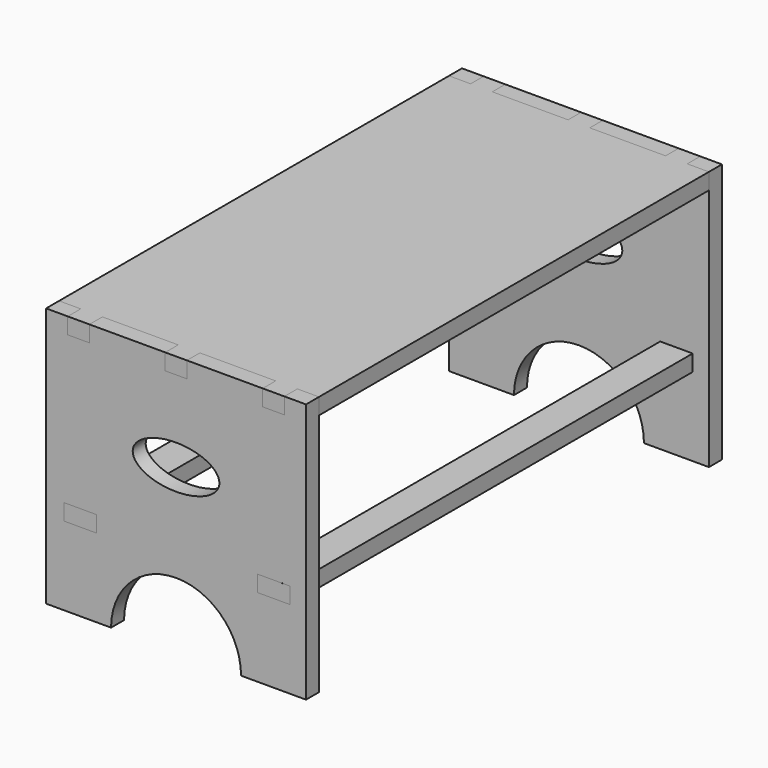
from build123d import *

# Parameters (mm, degrees)
F1_DEPTH = 19.05
F2_W     = 25.4
F2_H     = 19.05
F2_W_2   = 88.9
F3_DEPTH = 609.6
F2_W_3   = 38.1
F5_R     = 76.19999
F5_2_R   = 76.19999


# Not quite as in the source:
# - a fillet or chamfer is up to 0.001 mm smaller than in the source, because OpenCascade refuses the exact size


with BuildPart() as f1:
    # F0 (on Front) → F1 (new body)
    with BuildSketch(Plane.XZ):
        Polygon((0, 304.8), (0, 0), (76.2, 0), (76.2, 76.2), (228.6, 76.2), (228.6, 0), (304.8, 0), (304.8, 304.8), (279.4, 304.8), (279.4, 285.75), (254, 285.75), (254, 304.8), (165.1, 304.8), (165.1, 285.75), (139.7, 285.75), (139.7, 304.8), (50.8, 304.8), (50.8, 285.75), (25.4, 285.75), (25.4, 304.8), align=None)
        Polygon((59.3576016784, 92.0819193125), (53.0076016784, 92.0819193125), (27.6076016784, 92.0819193125), (25.4, 92.0819193125), (21.2576016784, 92.0819193125), (21.2576016784, 111.1319193125), (27.6076016784, 111.1319193125), (53.0076016784, 111.1319193125), (59.3576016784, 111.1319193125), align=None, mode=Mode.SUBTRACT)
        Polygon((254, 111.1180806875), (254, 111.1319193125), (279.4, 111.1319193125), (279.4, 111.1180806875), (285.75, 111.1180806875), (285.75, 92.0680806875), (279.4, 92.0680806875), (254, 92.0680806875), (247.65, 92.0680806875), (247.65, 111.1180806875), align=None, mode=Mode.SUBTRACT)
        with BuildLine():
            add(Edge.make_bspline(
                [(203.2, 190.5), (203.2, 234.4940905122), (127, 212.4970452561), (50.8, 190.5), (127, 168.5029547439), (203.2, 146.5059094878), (203.2, 190.5)],
                knots=[0, 0, 0, 2.0943951024, 2.0943951024, 4.1887902048, 4.1887902048, 6.2831853072, 6.2831853072, 6.2831853072], degree=2, weights=[1, 0.5, 1, 0.5, 1, 0.5, 1]))
        make_face(mode=Mode.SUBTRACT)
    extrude(amount=F1_DEPTH)


with BuildPart() as f3:
    # F2 (on face) → F3 (new body)
    with BuildSketch(Plane(origin=(0, 0, 0), x_dir=(-1, 0, 0), z_dir=(0, 1, 0))):
        with Locations((-292.1, 295.275)):
            Rectangle(F2_W, F2_H)
        with Locations((-266.7, 295.275)):
            Rectangle(F2_W, F2_H)
        with Locations((-209.55, 295.275)):
            Rectangle(F2_W_2, F2_H)
        with Locations((-152.4, 295.275)):
            Rectangle(F2_W, F2_H)
        with Locations((-95.25, 295.275)):
            Rectangle(F2_W_2, F2_H)
        with Locations((-38.1, 295.275)):
            Rectangle(F2_W, F2_H)
        with Locations((-12.7, 295.275)):
            Rectangle(F2_W, F2_H)
    extrude(amount=-F3_DEPTH)


with BuildPart() as f3b:
    # F2 (on face) → F3, piece 2 (new body)
    with BuildSketch(Plane(origin=(0, 0, 0), x_dir=(-1, 0, 0), z_dir=(0, 1, 0))):
        with Locations((-40.3076016784, 101.6069193125)):
            Rectangle(F2_W_3, F2_H)
    extrude(amount=-F3_DEPTH)


with BuildPart() as f3c:
    # F2 (on face) → F3, piece 3 (new body)
    with BuildSketch(Plane(origin=(0, 0, 0), x_dir=(-1, 0, 0), z_dir=(0, 1, 0))):
        Polygon((-247.65, 92.0680806875), (-247.65, 111.1180806875), (-254, 111.1180806875), (-279.4, 111.1180806875), (-285.75, 111.1180806875), (-285.75, 92.0680806875), align=None)
    extrude(amount=-F3_DEPTH)


with BuildPart() as f4_1:
    # F4: copy of F1
    add(f1.part.moved(Location((0, -590.55, 0))))

    # F5#2 (radius 76.2 in the source; OpenCascade refuses exactly that, so slightly less here)
    f5_2_edges = [f4_1.edges().sort_by_distance(p)[0] for p in [
        (228.6, -600.075, 76.2),
        (76.2, -600.075, 76.2),
    ]]
    fillet(f5_2_edges, radius=F5_2_R)


with BuildPart() as f1_1:
    add(f1.part)

    # F5 (radius 76.2 in the source; OpenCascade refuses exactly that, so slightly less here)
    f5_edges = [f1_1.edges().sort_by_distance(p)[0] for p in [
        (76.2, -9.525, 76.2),
        (228.6, -9.525, 76.2),
    ]]
    fillet(f5_edges, radius=F5_R)


with BuildPart() as f3_1:
    add(f3.part)

    # F6: cut F4_1
    add(f4_1.part, mode=Mode.SUBTRACT)

    # F7: cut F1
    add(f1_1.part, mode=Mode.SUBTRACT)


solid = Compound([f3b.part, f3c.part, f4_1.part, f1_1.part, f3_1.part])
